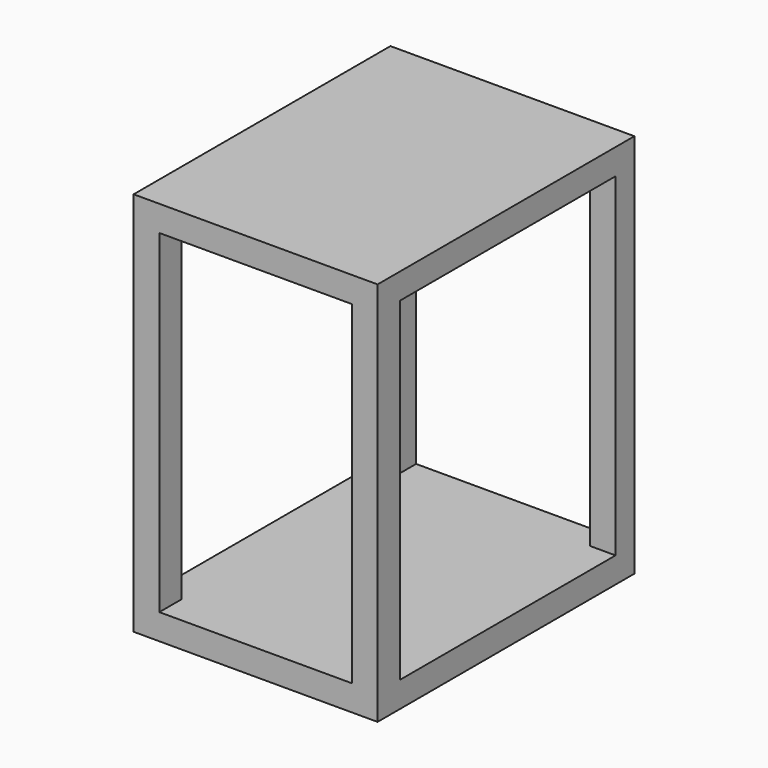
from build123d import *

# Parameters (mm, degrees)
F0_W     = 381
F0_H     = 50.8
F1_DEPTH = 635
F2_W     = 533.4
F2_H     = 660.4
F3_DEPTH = 482.601
F0_H_2   = 660.4
F4_DEPTH = 635.001


# Not quite as in the source:
# - a feature names something its author has since deleted; it is built from what else it names


with BuildPart() as f1:
    # F0 (on Front) → F1 (new body)
    with BuildSketch(Plane.XZ):
        with Locations((0, 355.6)):
            Rectangle(F0_W, F0_H)
        Polygon((241.3, 381), (190.5, 381), (190.5, 330.2), (190.5, -330.2), (190.5, -381), (241.3, -381), align=None)
        with Locations((0, -355.6)):
            Rectangle(F0_W, F0_H)
        Polygon((-190.5, 381), (-241.3, 381), (-241.3, -381), (-190.5, -381), (-190.5, -330.2), (-190.5, 330.2), align=None)
    extrude(amount=-F1_DEPTH)

    # F2 (on face) → F3 (cut, through all)
    with BuildSketch(Plane.YZ.offset(241.3)):
        with Locations((321.7956796288, 0)):
            Rectangle(F2_W, F2_H)
    extrude(amount=-F3_DEPTH, mode=Mode.SUBTRACT)

    # F0 (on Front) → F4 (cut, through all)
    with BuildSketch(Plane.XZ):
        Rectangle(F0_W, F0_H_2)
    extrude(amount=-F4_DEPTH, mode=Mode.SUBTRACT)


solid = f1.part
